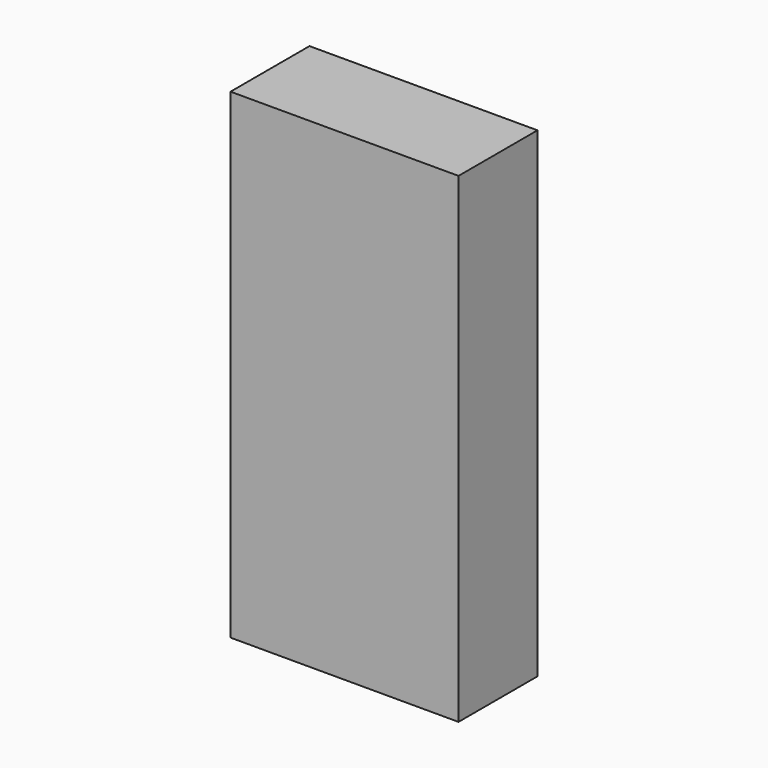
from build123d import *

# Parameters (mm, degrees)
F1_DEPTH = 25.4


# Not quite as in the source:
# - ends of sketch curves that miss each other by under 0.0002 mm in the source are joined


with BuildPart() as f1:
    # F0 (on Front) → F1 (new body)
    with BuildSketch(Plane.XZ):
        Polygon((58.674, 141.5296868842), (0, 141.5296868842), (0, 17.8316868842), (58.6739985928, 17.8188364873), align=None)
    extrude(amount=F1_DEPTH)


solid = f1.part
